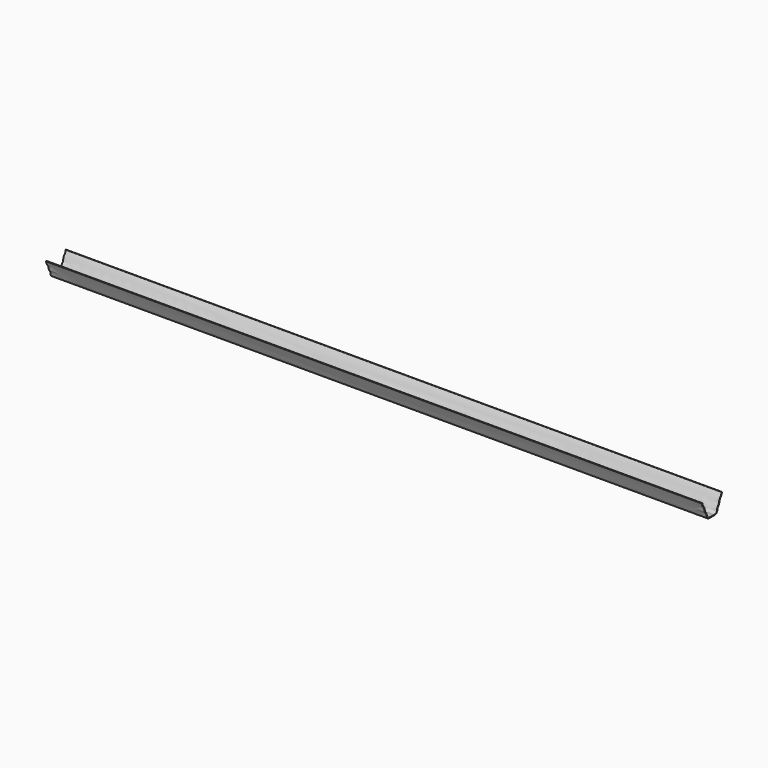
from build123d import *

# Parameters (mm, degrees)
F1_DEPTH = 3600


# Not quite as in the source:
# - ends of sketch curves that miss each other by under 0.0002 mm in the source are joined
# - the dataset's text gives a spline's control points without its knots; the knots are read off the source's solid


with BuildPart() as f1:
    # F0 (on Right) → F1 (new body)
    with BuildSketch(Plane.YZ):
        with BuildLine():
            add(Edge.make_bspline(
                [(-6.5371447453, 100.0838043479), (-6.7706498844, 98.7103560222), (-7.2769413201, 95.966442744), (-8.2462300011, 91.9595019059), (-9.3037510376, 88.7948658007), (-10.3440569893, 86.4178038959), (-11.2307456768, 84.7238978183), (-12.2403989924, 83.1327544504), (-13.7314030487, 81.0971306843), (-15.7697396376, 78.6342860816), (-17.8019003352, 76.0598448924), (-19.2697771779, 73.7976975728), (-20.2543484515, 71.9667309835), (-21.0728069506, 69.9675927938), (-21.9644751836, 67.1317082104), (-22.8208505479, 63.3393291587), (-23.5880679523, 59.4204357255), (-24.2982442677, 56.3341514977), (-24.9152930999, 54.0757040586), (-25.5299125954, 52.2670731086), (-26.0987925353, 50.8798986568), (-26.7265419191, 49.5377250168), (-27.6192869804, 47.9259926379), (-28.8144352862, 46.0694225719), (-30.0870954542, 44.2604615596), (-31.3889305982, 42.4695513152), (-32.6711410298, 40.6663234118), (-33.8840399285, 38.8197513275), (-34.9770680963, 36.8983087952), (-35.7441787823, 35.2087841297), (-36.245684668, 33.7892000703), (-36.6603912488, 32.3205401383), (-37.0314295875, 30.4232254421), (-37.3426701, 28.0880308878), (-37.7016109413, 24.956073947), (-38.2751198805, 21.1168701085), (-39.5879465674, 17.6919434206), (-41.4132093167, 15.3464026837), (-43.884361824, 13.3003757024), (-48.4648476434, 11.3486413482), (-54.6911472323, 10.0868951516), (-58.9601875507, 9.6146321059), (-60.5720902436, 9.4757778746)],
                knots=[0, 0, 0, 0, 0.03125, 0.0625, 0.09375, 0.109375, 0.125, 0.140625, 0.15625, 0.1875, 0.21875, 0.234375, 0.25, 0.265625, 0.28125, 0.3125, 0.34375, 0.359375, 0.375, 0.390625, 0.3984375, 0.40625, 0.421875, 0.4375, 0.453125, 0.46875, 0.484375, 0.5, 0.515625, 0.53125, 0.5390625, 0.546875, 0.5625, 0.578125, 0.59375, 0.625, 0.65625, 0.671875, 0.6875, 0.71875, 0.75, 0.7681993638, 0.7681993638, 0.7681993638, 0.7681993638], degree=3))
            ThreePointArc((-6.5371447453, 100.0838043479), (-7.7645113289, 101.8139967008), (-9.4947036818, 100.5866301172))
            add(Edge.make_bspline(
                [(-9.4947036818, 100.5866301172), (-9.723489658, 99.2409393238), (-10.2154650316, 96.5775155495), (-10.984099453, 93.4060678093), (-11.7253161057, 91.0179222177), (-12.351032201, 89.3152360524), (-12.9364195699, 87.9786891729), (-13.445069822, 86.9641431497), (-13.8449752198, 86.237110404), (-14.2714951974, 85.5325548459), (-14.883703547, 84.6020829341), (-15.7352720489, 83.4380223818), (-16.8740485904, 82.0050765428), (-18.0941724522, 80.5130147466), (-19.3606115163, 78.9279555444), (-20.4182743502, 77.4990743402), (-21.2400483814, 76.2738452745), (-21.8370919113, 75.3102683333), (-22.4086512808, 74.2972930377), (-22.9492281356, 73.2237773821), (-23.4401123128, 72.1063379574), (-24.0242674729, 70.5860968403), (-24.6327831857, 68.64688946), (-25.2296829702, 66.2937826991), (-25.7451190854, 63.9292340336), (-26.2217625213, 61.5819904015), (-26.6985692792, 59.280556009), (-27.2107834687, 57.056451861), (-27.6926120569, 55.295580755), (-28.1236953584, 53.960179636), (-28.473009584, 52.9974452444), (-28.8479928364, 52.0836294372), (-29.3934828733, 50.9171718759), (-30.1894656071, 49.4774115594), (-31.2965609822, 47.7557860025), (-32.5198063414, 46.0161067231), (-33.8170759051, 44.2313930138), (-35.140653965, 42.37078801), (-36.43738975, 40.3984692762), (-37.4456660647, 38.6286705807), (-38.1730927218, 37.1189779146), (-38.5863632984, 36.1338877597), (-38.8873866246, 35.3191685524), (-39.0976860325, 34.6916248477), (-39.2882860981, 34.0554206664), (-39.5152977744, 33.2063939821), (-39.7518092025, 32.1482507218), (-40.0512888446, 30.478702112), (-40.3223470736, 28.4366280651), (-40.5908821572, 26.094352671), (-40.89399031, 23.9016800338), (-41.3011875448, 21.9112530753), (-41.8613191997, 20.1758141026), (-42.6066042503, 18.7044565974), (-43.4154210799, 17.6672121122), (-44.2460282782, 16.9035328467), (-44.9853969828, 16.3577743125), (-45.8907269157, 15.8235872099), (-46.9721354151, 15.3045309126), (-48.2104811138, 14.8152141046), (-50.0529843689, 14.2110000128), (-52.6812922381, 13.5577191822), (-56.2490599407, 12.9455882658), (-59.0331081681, 12.6252377637), (-60.5727693793, 12.4869516331), (-60.7761499105, 12.4693210267)],
                knots=[0, 0, 0, 0, 0.03125, 0.0625, 0.078125, 0.09375, 0.109375, 0.1171875, 0.125, 0.1328125, 0.140625, 0.15625, 0.171875, 0.1875, 0.203125, 0.21875, 0.2265625, 0.234375, 0.2421875, 0.25, 0.2578125, 0.265625, 0.28125, 0.296875, 0.3125, 0.328125, 0.34375, 0.359375, 0.375, 0.3828125, 0.390625, 0.3984375, 0.40625, 0.421875, 0.4375, 0.453125, 0.46875, 0.484375, 0.5, 0.515625, 0.5234375, 0.53125, 0.53515625, 0.5390625, 0.54296875, 0.546875, 0.5546875, 0.5625, 0.578125, 0.59375, 0.609375, 0.625, 0.640625, 0.65625, 0.671875, 0.6796875, 0.6875, 0.6953125, 0.703125, 0.7109375, 0.71875, 0.734375, 0.75, 0.765625, 0.7679922272, 0.7679922272, 0.7679922272, 0.7679922272], degree=3))
            add(Edge.make_bspline(
                [(-140.5052963182, 100.5866301172), (-140.276510342, 99.2409393238), (-139.7845349684, 96.5775155495), (-139.015900547, 93.4060678093), (-138.2746838943, 91.0179222177), (-137.648967799, 89.3152360524), (-137.0635804301, 87.9786891729), (-136.554930178, 86.9641431497), (-136.1550247802, 86.237110404), (-135.7285048026, 85.5325548459), (-135.116296453, 84.6020829341), (-134.2647279511, 83.4380223818), (-133.1259514096, 82.0050765428), (-131.9058275478, 80.5130147466), (-130.6393884837, 78.9279555444), (-129.5817256498, 77.4990743402), (-128.7599516186, 76.2738452745), (-128.1629080887, 75.3102683333), (-127.5913487192, 74.2972930377), (-127.0507718644, 73.2237773821), (-126.5598876872, 72.1063379574), (-125.9757325271, 70.5860968403), (-125.3672168143, 68.64688946), (-124.7703170298, 66.2937826991), (-124.2548809146, 63.9292340336), (-123.7782374787, 61.5819904015), (-123.3014307208, 59.280556009), (-122.7892165313, 57.056451861), (-122.3073879431, 55.295580755), (-121.8763046416, 53.960179636), (-121.526990416, 52.9974452444), (-121.1520071636, 52.0836294372), (-120.6065171267, 50.9171718759), (-119.8105343929, 49.4774115594), (-118.7034390178, 47.7557860025), (-117.4801936586, 46.0161067231), (-116.1829240949, 44.2313930138), (-114.859346035, 42.37078801), (-113.56261025, 40.3984692762), (-112.5543339353, 38.6286705807), (-111.8269072782, 37.1189779146), (-111.4136367016, 36.1338877597), (-111.1126133754, 35.3191685524), (-110.9023139675, 34.6916248477), (-110.7117139019, 34.0554206664), (-110.4847022256, 33.2063939821), (-110.2481907975, 32.1482507218), (-109.9487111554, 30.478702112), (-109.6776529264, 28.4366280651), (-109.4091178428, 26.094352671), (-109.10600969, 23.9016800338), (-108.6988124552, 21.9112530753), (-108.1386808003, 20.1758141026), (-107.3933957497, 18.7044565974), (-106.5845789201, 17.6672121122), (-105.7539717218, 16.9035328467), (-105.0146030172, 16.3577743125), (-104.1092730843, 15.8235872099), (-103.0278645849, 15.3045309126), (-101.7895188862, 14.8152141046), (-99.9470156311, 14.2110000128), (-97.3187077619, 13.5577191822), (-93.7509400593, 12.9455882658), (-89.8689345695, 12.4988997366), (-84.3935825665, 12.1034311284), (-77.2067630007, 11.9388633447), (-70.1126435589, 12.0750053269), (-64.809324713, 12.2759728551), (-62.201228655, 12.398488893), (-60.9005172536, 12.4631129163), (-60.7761499105, 12.4693210267)],
                knots=[0, 0, 0, 0, 0.03125, 0.0625, 0.078125, 0.09375, 0.109375, 0.1171875, 0.125, 0.1328125, 0.140625, 0.15625, 0.171875, 0.1875, 0.203125, 0.21875, 0.2265625, 0.234375, 0.2421875, 0.25, 0.2578125, 0.265625, 0.28125, 0.296875, 0.3125, 0.328125, 0.34375, 0.359375, 0.375, 0.3828125, 0.390625, 0.3984375, 0.40625, 0.421875, 0.4375, 0.453125, 0.46875, 0.484375, 0.5, 0.515625, 0.5234375, 0.53125, 0.53515625, 0.5390625, 0.54296875, 0.546875, 0.5546875, 0.5625, 0.578125, 0.59375, 0.609375, 0.625, 0.640625, 0.65625, 0.671875, 0.6796875, 0.6875, 0.6953125, 0.703125, 0.7109375, 0.71875, 0.734375, 0.75, 0.765625, 0.78125, 0.8125, 0.84375, 0.859375, 0.875, 0.8766615277, 0.8766615277, 0.8766615277, 0.8766615277], degree=3))
            ThreePointArc((-140.5052963182, 100.5866301172), (-142.2354886711, 101.8139967008), (-143.4628552547, 100.0838043479))
            add(Edge.make_bspline(
                [(-143.4628552547, 100.0838043479), (-143.2293501156, 98.7103560222), (-142.7230586799, 95.966442744), (-141.7537699989, 91.9595019059), (-140.6962489624, 88.7948658007), (-139.6559430107, 86.4178038959), (-138.7692543232, 84.7238978183), (-137.7596010076, 83.1327544504), (-136.2685969513, 81.0971306843), (-134.2302603624, 78.6342860816), (-132.1980996648, 76.0598448924), (-130.7302228221, 73.7976975728), (-129.7456515485, 71.9667309835), (-128.9271930494, 69.9675927938), (-128.0355248164, 67.1317082104), (-127.1791494521, 63.3393291587), (-126.4119320477, 59.4204357255), (-125.7017557323, 56.3341514977), (-125.0847069001, 54.0757040586), (-124.4700874046, 52.2670731086), (-123.9012074647, 50.8798986568), (-123.2734580809, 49.5377250168), (-122.3807130196, 47.9259926379), (-121.1855647138, 46.0694225719), (-119.9129045458, 44.2604615596), (-118.6110694018, 42.4695513152), (-117.3288589702, 40.6663234118), (-116.1159600715, 38.8197513275), (-115.0229319037, 36.8983087952), (-114.2558212177, 35.2087841297), (-113.754315332, 33.7892000703), (-113.3396087512, 32.3205401383), (-112.9685704125, 30.4232254421), (-112.6573299, 28.0880308878), (-112.2983890587, 24.956073947), (-111.7248801195, 21.1168701085), (-110.4120534326, 17.6919434206), (-108.5867906833, 15.3464026837), (-106.115638176, 13.3003757024), (-101.5351523566, 11.3486413482), (-94.301940604, 9.8828465711), (-85.9812891212, 9.1380434831), (-77.2034138309, 8.9381010647), (-70.0276489837, 9.0760424081), (-64.6807378705, 9.2786910878), (-62.0382645593, 9.4028348724), (-60.7148909827, 9.4686377045), (-60.5720902436, 9.4757778746)],
                knots=[0, 0, 0, 0, 0.03125, 0.0625, 0.09375, 0.109375, 0.125, 0.140625, 0.15625, 0.1875, 0.21875, 0.234375, 0.25, 0.265625, 0.28125, 0.3125, 0.34375, 0.359375, 0.375, 0.390625, 0.3984375, 0.40625, 0.421875, 0.4375, 0.453125, 0.46875, 0.484375, 0.5, 0.515625, 0.53125, 0.5390625, 0.546875, 0.5625, 0.578125, 0.59375, 0.625, 0.65625, 0.671875, 0.6875, 0.71875, 0.75, 0.78125, 0.8125, 0.84375, 0.859375, 0.875, 0.8769032209, 0.8769032209, 0.8769032209, 0.8769032209], degree=3))
        make_face()
    extrude(amount=F1_DEPTH)


solid = f1.part
